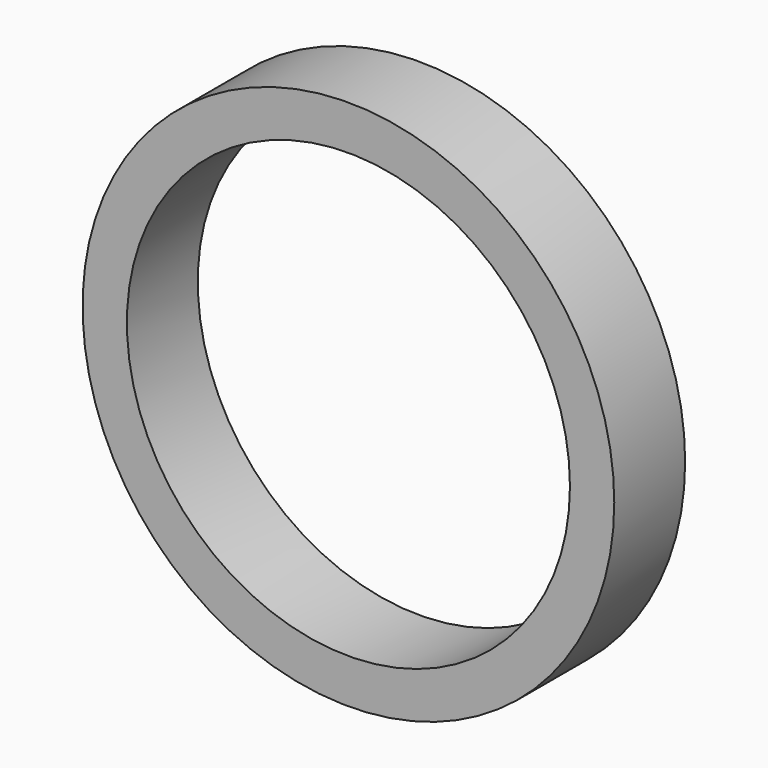
from build123d import *

# Parameters (mm, degrees)
F0_R     = 30.48
F0_R_2   = 27.94
F0_R_3   = 25.4
F1_DEPTH = 10.16


# Not quite as in the source:
# - a feature of the source that left no trace in its solid (it failed there, or was rolled back) is left out


with BuildPart() as f1:
    # F0 (on Front) → F1 (new body)
    with BuildSketch(Plane.XZ):
        Circle(F0_R)
        Circle(F0_R_2, mode=Mode.SUBTRACT)
        Circle(F0_R_2)
        Circle(F0_R_3, mode=Mode.SUBTRACT)
    extrude(amount=F1_DEPTH)


solid = f1.part
